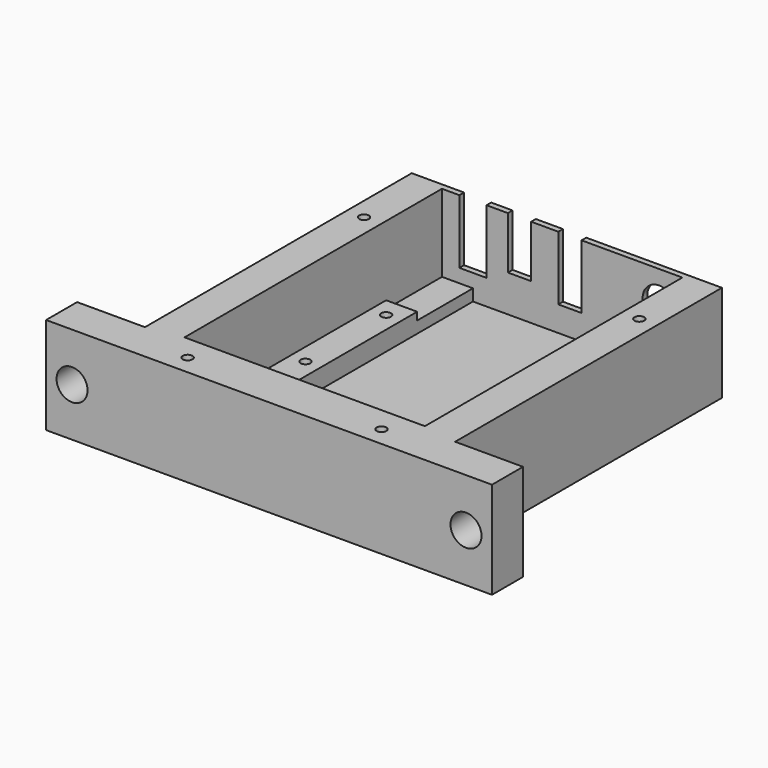
from build123d import *

# Parameters (mm, degrees)
F1_DEPTH  = 25
F2_W      = 62
F2_H      = 83
F3_DEPTH  = 18
F4_W      = 46
F4_H      = 83
F5_DEPTH  = 5
F7_D      = 2.5
F7_DEPTH  = 5.5
F7_TIP    = 0.7510757738
F8_W      = 62
F8_H      = 15
F9_DEPTH  = 25.001
F11_D     = 8
F12_W     = 6
F12_H     = 16.5
F12_H_2   = 13.5
F12_W_2   = 7
F13_DEPTH = 1.5
F14_W     = 8
F14_H     = 18
F15_DEPTH = 2
F16_R     = 4.25
F17_DEPTH = 1.5
F18_W     = 5
F18_H     = 0.7
F19_DEPTH = 5
F21_D     = 2.5
F21_DEPTH = 7
F21_TIP   = 0.7510757738


# Not quite as in the source:
# - a pattern or mirror of a feature is missing from the dataset's text; its kind, count and spacing are read off the source's solid


with BuildPart() as f1:
    # F0 (on Top) → F1 (new body)
    with BuildSketch(Plane.XY):
        Polygon((40, 48), (-40, 48), (-40, -38), (-57.5, -38), (-57.5, -48), (57.5, -48), (57.5, -38), (40, -38), align=None)
    extrude(amount=F1_DEPTH)

    # F2 (on face) → F3 (cut)
    with BuildSketch(Plane.XY.offset(25)):
        with Locations((0, 5)):
            Rectangle(F2_W, F2_H)
    extrude(amount=-F3_DEPTH, mode=Mode.SUBTRACT)

    # F4 (on face) → F5 (cut)
    with BuildSketch(Plane.XY.offset(7)):
        with Locations((0, 5)):
            Rectangle(F4_W, F4_H)
    extrude(amount=-F5_DEPTH, mode=Mode.SUBTRACT)

    # F7
    with Locations(Plane.XY.offset(7)):
        with Locations((-27, -32.5), (-27, -2.5), (-27, 23.5), (27, -32.5), (27, -2.5), (27, 23.5)):
            Hole(F7_D / 2, depth=F7_DEPTH)
            with Locations((0, 0, -(F7_DEPTH + F7_TIP / 2))):  # 118° drill point
                Cone(0, F7_D / 2, F7_TIP, mode=Mode.SUBTRACT)

    # F8 (on face) → F9 (cut, through all)
    with BuildSketch(Plane(origin=(0, 0, 0), x_dir=(1, 0, 0), z_dir=(0, 0, -1))):
        with Locations((0, 17.5)):
            Rectangle(F8_W, F8_H)
    extrude(amount=-F9_DEPTH, mode=Mode.SUBTRACT)

    # F11 (through all)
    with Locations(Plane(origin=(0, -38, 0), x_dir=(-1, 0, 0), z_dir=(0, 1, 0))):
        with Locations((50.8, 12.5), (-50.8, 12.5)):
            Hole(F11_D / 2)

    # F12 (on face) → F13 (cut, through all)
    with BuildSketch(Plane(origin=(0, 48, 0), x_dir=(-1, 0, 0), z_dir=(0, 1, 0))):
        with Locations((-2, 16.75)):
            Rectangle(F12_W, F12_H)
        with Locations((11, 18.25)):
            Rectangle(F12_W, F12_H_2)
        with Locations((23, 16.75)):
            Rectangle(F12_W_2, F12_H)
    extrude(amount=-F13_DEPTH, mode=Mode.SUBTRACT)

    # F14 (on face) → F15 (cut)
    with BuildSketch(Plane.XY.offset(7)):
        with Locations((-27, 37.5)):
            Rectangle(F14_W, F14_H)
    extrude(amount=-F15_DEPTH, mode=Mode.SUBTRACT)

    # F16 (on face) → F17 (cut, through all)
    with BuildSketch(Plane(origin=(0, 48, 0), x_dir=(-1, 0, 0), z_dir=(0, 1, 0))):
        with Locations((-25, 17)):
            Circle(F16_R)
    extrude(amount=-F17_DEPTH, mode=Mode.SUBTRACT)

    # F18 (on face) → F19 (cut)
    with BuildSketch(Plane.YZ.offset(40)):
        with Locations((-35.5, 0.35)):
            Rectangle(F18_W, F18_H)
    f19 = extrude(amount=-F19_DEPTH, mode=Mode.SUBTRACT)

    # F19_copies: F19 across plane
    add(f19.mirror(Plane(origin=(0, 0, 0), x_dir=(0, 0, -1), z_dir=(-1, 0, 0))), mode=Mode.SUBTRACT)

    # F21
    with Locations(Plane.XY.offset(25)):
        with Locations((25, -43), (-25, -43), (35.5, 27), (-35.5, 27)):
            Hole(F21_D / 2, depth=F21_DEPTH)
            with Locations((0, 0, -(F21_DEPTH + F21_TIP / 2))):  # 118° drill point
                Cone(0, F21_D / 2, F21_TIP, mode=Mode.SUBTRACT)


solid = f1.part
